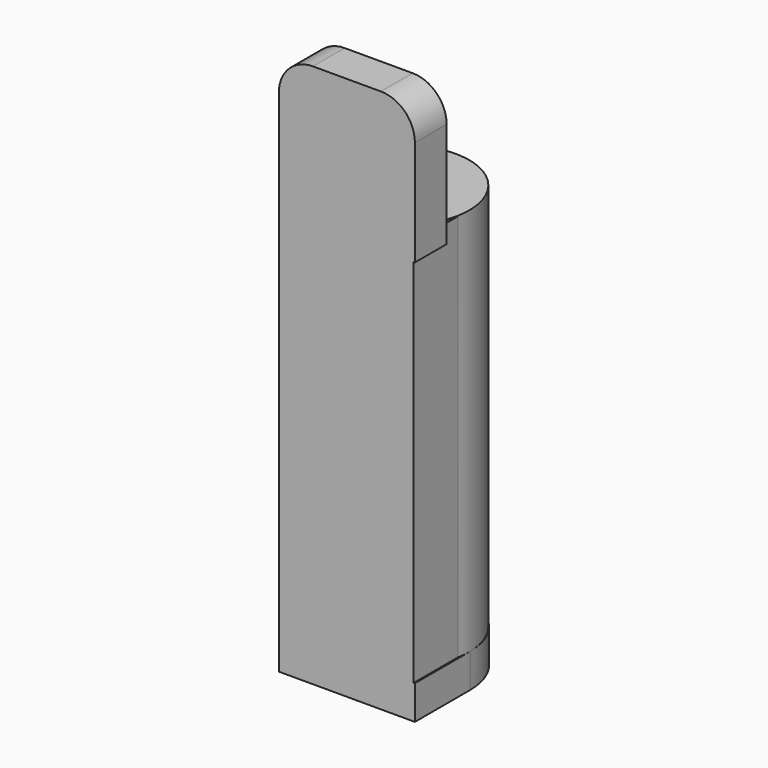
from build123d import *

# Parameters (mm, degrees)
F0_R        = 6
F1_DEPTH    = 37.3
F2_W        = 12
F2_H        = 12
F3_DEPTH    = 3
F4_W        = 12
F4_H        = 12.3061701586
F5_DEPTH    = 3.5
F6_W        = 2
F6_H        = 10
F7_DEPTH    = 6
F8_T1_DEPTH = 32.5803989155
F9_W        = 11.8940497642
F9_H        = 34.25
F10_DEPTH   = 6
F11_R       = 2.25
F12_DEPTH   = 34.3
F13_R       = 3


# Not quite as in the source:
# - a fillet or chamfer that OpenCascade refuses, or shapes differently, is made with other operations: its cross-section is extruded or revolved along the edge and cut away or added


with BuildPart() as f1:
    # F0 (on Top) → F1 (new body)
    with BuildSketch(Plane.XY):
        Circle(F0_R)
    extrude(amount=F1_DEPTH)

    # F2 (on face) → F3 (join)
    with BuildSketch(Plane(origin=(0, 0, 0), x_dir=(1, 0, 0), z_dir=(0, 0, -1))):
        Rectangle(F2_W, F2_H)
    extrude(amount=-F3_DEPTH)

    # F4 (on face) → F5 (join)
    with BuildSketch(Plane.XZ.offset(6)):
        with Locations((0, 41.8383553624)):
            Rectangle(F4_W, F4_H)
    extrude(amount=-F5_DEPTH)

    # F6 (on face) → F7 (cut)
    with BuildSketch(Plane(origin=(0, 6, 0), x_dir=(-1, 0, 0), z_dir=(0, 1, 0))):
        with Locations((0, 5)):
            Rectangle(F6_W, F6_H)
    extrude(amount=-F7_DEPTH, mode=Mode.SUBTRACT)

    # F8: fillet of radius 6 on 2 edges, made by hand

    # F8_s2 → F8_t1 (cut)
    with BuildSketch(Plane.XY.offset(-14.7901994578)):
        with BuildLine():
            ThreePointArc((-1, 6), (-4.582575695, 3.9569035631), (-6, 0.0839202169))
            Line((-6, 0.0839202169), (-6, 6))
            Line((-6, 6), (-1, 6))
        make_face()
        with BuildLine():
            ThreePointArc((1, 6), (4.582575695, 3.9569035631), (6, 0.0839202169))
            Line((6, 0.0839202169), (6, 6))
            Line((6, 6), (1, 6))
        make_face()
    extrude(amount=F8_T1_DEPTH, mode=Mode.SUBTRACT)

    # F9 (on face) → F10 (join)
    with BuildSketch(Plane.XZ.offset(6)):
        with Locations((-0.0529751179, 20.125)):
            Rectangle(F9_W, F9_H)
    extrude(amount=-F10_DEPTH)

    # F11 (on face) → F12 (cut)
    with BuildSketch(Plane.XY.offset(37.3)):
        Circle(F11_R)
    extrude(amount=-F12_DEPTH, mode=Mode.SUBTRACT)

    # F13
    f13_edges = [f1.edges().sort_by_distance(p)[0] for p in [
        (6, -4.25, 47.99144),
        (-6, -4.25, 47.99144),
    ]]
    fillet(f13_edges, radius=F13_R)


solid = f1.part
